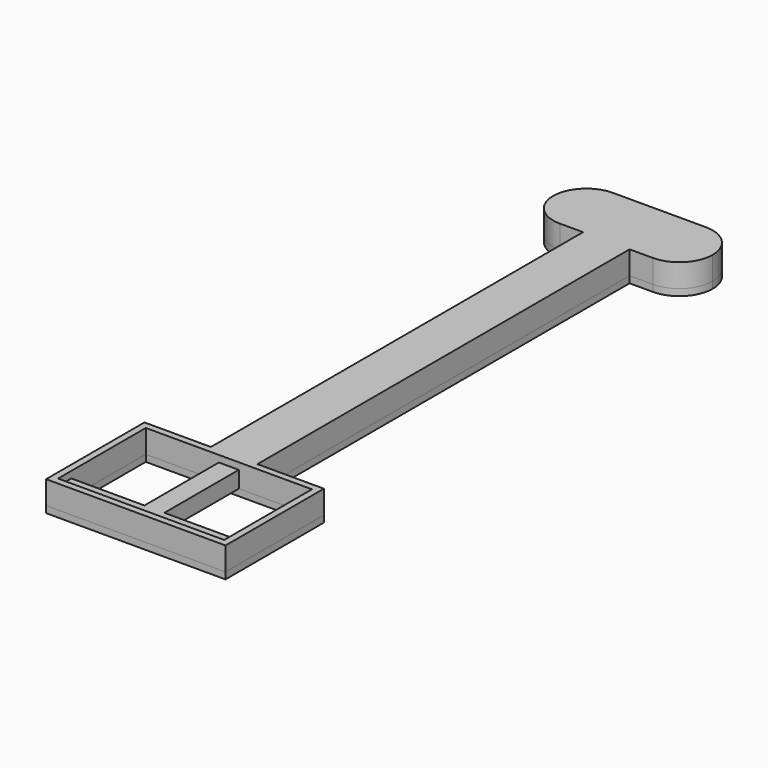
from build123d import *

# Parameters (mm, degrees)
F1_DEPTH      = 5
F3_W          = 22
F3_H          = 5
F3_W_2        = 6
F4_DEPTH      = 5
F5_W          = 50
F5_H          = 33
F6_DEPTH      = 7
F6_DEPTH_BACK = 2


with BuildPart() as f1:
    # F0 (on Top) → F1 (new body)
    with BuildSketch(Plane.XY):
        Polygon((3, 13), (0, 13), (0, -180), (3, -180), (3, -39.0871235167), (3, -36.9128764833), (3, -35.8871235167), (3, -33.7128764833), (3, -32.6871235167), (3, -30.5128764833), (3, -29.4871235167), (3, -27.3128764833), (3, -26.2871235167), (3, -24.1128764833), (3, -23.0871235167), (3, -20.9128764833), (3, -19.8871235167), (3, -17.7128764833), (3, -16.6871235167), (3, -14.5128764833), (3, -13.4871235167), (3, -11.3128764833), (3, -10.2871235167), (3, -8.1128764833), (3, -7.0871235167), (3, -4.9128764833), (3, -3.8871235167), (3, -1.7128764833), (3, -0.6871235167), (3, 1.4871235167), (3, 2.5128764833), (3, 4.6871235167), (3, 5.7128764833), (3, 7.8871235167), (3, 8.9128764833), (3, 11.0871235167), align=None)
        with BuildLine():
            Line((3, -36.9128764833), (3, -39.0871235167))
            ThreePointArc((3, -39.0871235167), (4.0421988802, -38.9373096378), (5, -38.5))
            Line((5, -38.5), (5, -38))
            Line((5, -38), (5, -37.5))
            ThreePointArc((5, -37.5), (4.0421988802, -37.0626903622), (3, -36.9128764833))
        make_face()
        with BuildLine():
            Line((3, -33.7128764833), (3, -35.8871235167))
            ThreePointArc((3, -35.8871235167), (4.0421988802, -35.7373096378), (5, -35.3))
            Line((5, -35.3), (5, -34.8))
            Line((5, -34.8), (5, -34.3))
            ThreePointArc((5, -34.3), (4.0421988802, -33.8626903622), (3, -33.7128764833))
        make_face()
        with BuildLine():
            Line((3, -30.5128764833), (3, -32.6871235167))
            ThreePointArc((3, -32.6871235167), (4.0421988802, -32.5373096378), (5, -32.1))
            Line((5, -32.1), (5, -31.6))
            Line((5, -31.6), (5, -31.1))
            ThreePointArc((5, -31.1), (4.0421988802, -30.6626903622), (3, -30.5128764833))
        make_face()
        with BuildLine():
            Line((3, -27.3128764833), (3, -29.4871235167))
            ThreePointArc((3, -29.4871235167), (4.0421988802, -29.3373096378), (5, -28.9))
            Line((5, -28.9), (5, -28.4))
            Line((5, -28.4), (5, -27.9))
            ThreePointArc((5, -27.9), (4.0421988802, -27.4626903622), (3, -27.3128764833))
        make_face()
        with BuildLine():
            Line((3, -24.1128764833), (3, -26.2871235167))
            ThreePointArc((3, -26.2871235167), (4.0421988802, -26.1373096378), (5, -25.7))
            Line((5, -25.7), (5, -25.2))
            Line((5, -25.2), (5, -24.7))
            ThreePointArc((5, -24.7), (4.0421988802, -24.2626903622), (3, -24.1128764833))
        make_face()
        with BuildLine():
            Line((3, -20.9128764833), (3, -23.0871235167))
            ThreePointArc((3, -23.0871235167), (4.0421988802, -22.9373096378), (5, -22.5))
            Line((5, -22.5), (5, -22))
            Line((5, -22), (5, -21.5))
            ThreePointArc((5, -21.5), (4.0421988802, -21.0626903622), (3, -20.9128764833))
        make_face()
        with BuildLine():
            Line((3, -17.7128764833), (3, -19.8871235167))
            ThreePointArc((3, -19.8871235167), (4.0421988802, -19.7373096378), (5, -19.3))
            Line((5, -19.3), (5, -18.8))
            Line((5, -18.8), (5, -18.3))
            ThreePointArc((5, -18.3), (4.0421988802, -17.8626903622), (3, -17.7128764833))
        make_face()
        with BuildLine():
            Line((3, -14.5128764833), (3, -16.6871235167))
            ThreePointArc((3, -16.6871235167), (4.0421988802, -16.5373096378), (5, -16.1))
            Line((5, -16.1), (5, -15.6))
            Line((5, -15.6), (5, -15.1))
            ThreePointArc((5, -15.1), (4.0421988802, -14.6626903622), (3, -14.5128764833))
        make_face()
        with BuildLine():
            ThreePointArc((5, -11.9), (4.0421988802, -11.4626903622), (3, -11.3128764833))
            Line((3, -11.3128764833), (3, -13.4871235167))
            ThreePointArc((3, -13.4871235167), (4.0421988802, -13.3373096378), (5, -12.9))
            Line((5, -12.9), (5, -12.4))
            Line((5, -12.4), (5, -11.9))
        make_face()
        with BuildLine():
            ThreePointArc((5, -8.7), (4.0421988802, -8.2626903622), (3, -8.1128764833))
            Line((3, -8.1128764833), (3, -10.2871235167))
            ThreePointArc((3, -10.2871235167), (4.0421988802, -10.1373096378), (5, -9.7))
            Line((5, -9.7), (5, -9.2))
            Line((5, -9.2), (5, -8.7))
        make_face()
        with BuildLine():
            ThreePointArc((5, -5.5), (4.0421988802, -5.0626903622), (3, -4.9128764833))
            Line((3, -4.9128764833), (3, -7.0871235167))
            ThreePointArc((3, -7.0871235167), (4.0421988802, -6.9373096378), (5, -6.5))
            Line((5, -6.5), (5, -6))
            Line((5, -6), (5, -5.5))
        make_face()
        with BuildLine():
            ThreePointArc((5, -2.3), (4.0421988802, -1.8626903622), (3, -1.7128764833))
            Line((3, -1.7128764833), (3, -3.8871235167))
            ThreePointArc((3, -3.8871235167), (4.0421988802, -3.7373096378), (5, -3.3))
            Line((5, -3.3), (5, -2.8))
            Line((5, -2.8), (5, -2.3))
        make_face()
        with BuildLine():
            ThreePointArc((5, 0.9), (4.0421988802, 1.3373096378), (3, 1.4871235167))
            Line((3, 1.4871235167), (3, -0.6871235167))
            ThreePointArc((3, -0.6871235167), (4.0421988802, -0.5373096378), (5, -0.1))
            Line((5, -0.1), (5, 0.4))
            Line((5, 0.4), (5, 0.9))
        make_face()
        with BuildLine():
            ThreePointArc((5, 4.1), (4.0421988802, 4.5373096378), (3, 4.6871235167))
            Line((3, 4.6871235167), (3, 2.5128764833))
            ThreePointArc((3, 2.5128764833), (4.0421988802, 2.6626903622), (5, 3.1))
            Line((5, 3.1), (5, 3.6))
            Line((5, 3.6), (5, 4.1))
        make_face()
        with BuildLine():
            ThreePointArc((5, 7.3), (4.0421988802, 7.7373096378), (3, 7.8871235167))
            Line((3, 7.8871235167), (3, 5.7128764833))
            ThreePointArc((3, 5.7128764833), (4.0421988802, 5.8626903622), (5, 6.3))
            Line((5, 6.3), (5, 6.8))
            Line((5, 6.8), (5, 7.3))
        make_face()
        with BuildLine():
            ThreePointArc((5, 10.5), (4.0421988802, 10.9373096378), (3, 11.0871235167))
            Line((3, 11.0871235167), (3, 8.9128764833))
            ThreePointArc((3, 8.9128764833), (4.0421988802, 9.0626903622), (5, 9.5))
            Line((5, 9.5), (5, 10))
            Line((5, 10), (5, 10.5))
        make_face()
    extrude(amount=F1_DEPTH)

    # F2: F1 across face


with BuildPart() as f1_1:
    add(f1.part)
    add(f1.part.mirror(Plane(origin=(0, -83.5, 2.5), x_dir=(0, -1, 0), z_dir=(-1, 0, 0))))

    # F3 (on face) → F4 (join)
    with BuildSketch(Plane.XZ.offset(180)):
        with Locations((14, 2.5)):
            Rectangle(F3_W, F3_H)
        with Locations((0, 2.5)):
            Rectangle(F3_W_2, F3_H)
        with Locations((-14, 2.5)):
            Rectangle(F3_W, F3_H)
    extrude(amount=F4_DEPTH)


with BuildPart() as f6:
    # F5 (on Top) → F6 (new body, two sides)
    with BuildSketch(Plane.XY) as f6_sk:
        with BuildLine():
            ThreePointArc((14, -10), (4, 0), (14, 10))
            Line((14, 10), (0, 10))
            Line((0, 10), (-14, 10))
            ThreePointArc((-14, 10), (-6.9289321881, 7.0710678119), (-4, 0))
            ThreePointArc((-4, 0), (-6.9289321881, -7.0710678119), (-14, -10))
            Line((-14, -10), (-7, -10))
            Line((-7, -10), (-7, -150))
            Line((-7, -150), (-27, -150))
            Line((-27, -150), (-27, -187))
            Line((-27, -187), (0, -187))
            Line((0, -187), (27, -187))
            Line((27, -187), (27, -150))
            Line((27, -150), (7, -150))
            Line((7, -150), (7, -10))
            Line((7, -10), (14, -10))
        make_face()
        with Locations((0, -168.5)):
            Rectangle(F5_W, F5_H, mode=Mode.SUBTRACT)
        with BuildLine():
            ThreePointArc((-4, 0), (-6.9289321881, 7.0710678119), (-14, 10))
            ThreePointArc((-14, 10), (-24, 0), (-14, -10))
            ThreePointArc((-14, -10), (-6.9289321881, -7.0710678119), (-4, 0))
        make_face()
        with BuildLine():
            ThreePointArc((14, -10), (21.0710678119, -7.0710678119), (24, 0))
            ThreePointArc((24, 0), (21.0710678119, 7.0710678119), (14, 10))
            ThreePointArc((14, 10), (4, 0), (14, -10))
        make_face()
    extrude(amount=F6_DEPTH)
    extrude(f6_sk.sketch, amount=-F6_DEPTH_BACK)

    # F7: cut F1
    add(f1_1.part, mode=Mode.SUBTRACT)


solid = Compound([f1_1.part, f6.part])
